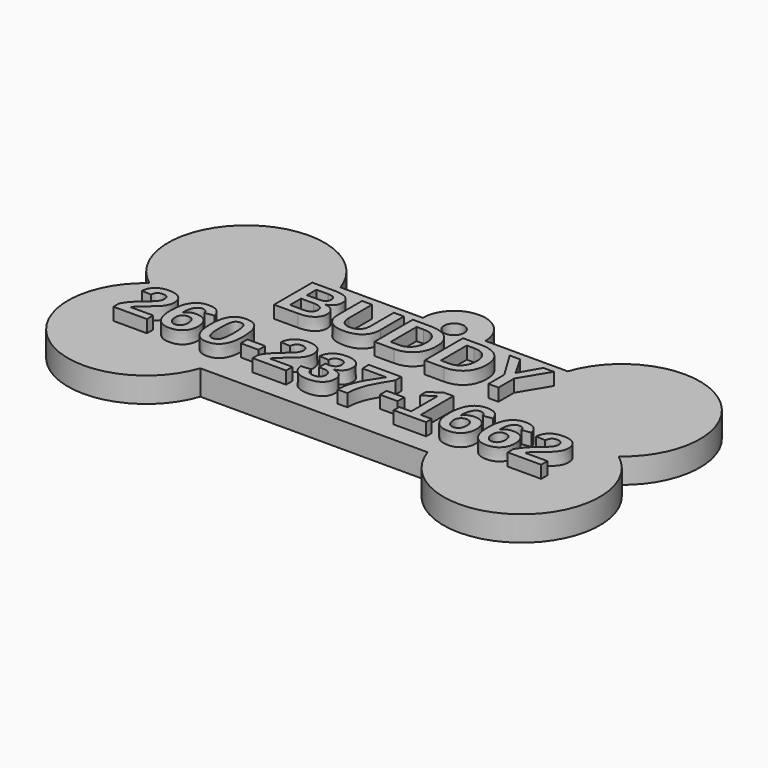
from build123d import *

# Parameters (mm, degrees)
F0_R         = 1.016
F1_DEPTH     = 2.54
F2_TEXT_SIZE = 7.0555555556
F3_DEPTH     = 1.27
F4_TEXT_SIZE = 7.0555555556
F5_DEPTH     = 1.27


# Not quite as in the source:
# - Text() gives the source's letters only with a copy of the font that has no kerning and outlines rounded to 1/6400 em; it was checked with that copy


with BuildPart() as f1:
    # F0 (on Top) → F1 (new body)
    with BuildSketch(Plane.XY):
        with BuildLine():
            Line((-15.2811150611, 27.291036626), (-23.6359883168, 27.291036626))
            ThreePointArc((-23.6359883168, 27.291036626), (-35.8100543941, 31.1810253456), (-35.9186150611, 18.401036626))
            ThreePointArc((-35.9186150611, 18.401036626), (-35.8100543941, 5.6210479063), (-23.6359883168, 9.511036626))
            Line((-23.6359883168, 9.511036626), (-0.5762418054, 9.511036626))
            ThreePointArc((-0.5762418054, 9.511036626), (11.5978242719, 5.6210479063), (11.7063849389, 18.401036626))
            ThreePointArc((11.7063849389, 18.401036626), (11.5978242719, 31.1810253456), (-0.5762418054, 27.291036626))
            Line((-0.5762418054, 27.291036626), (-8.9311150611, 27.291036626))
            ThreePointArc((-8.9311150611, 27.291036626), (-12.1061150611, 30.466036626), (-15.2811150611, 27.291036626))
        make_face()
        with Locations((-12.1061150611, 27.291036626)):
            Circle(F0_R, mode=Mode.SUBTRACT)
    extrude(amount=-F1_DEPTH)

    # F2 (on face) → F3 (join)
    with BuildSketch(Plane.XY):
        with Locations((-24.8380855472, 19.781898944)):
            Text('BUDDY', F2_TEXT_SIZE, font='Arimo', font_style=FontStyle.BOLD, text_align=(TextAlign.LEFT, TextAlign.BOTTOM))
    extrude(amount=F3_DEPTH)

    # F4 (on face) → F5 (join)
    with BuildSketch(Plane.XY):
        with Locations((-34.3300638513, 11.5541539654)):
            Text('260-237-1662', F4_TEXT_SIZE, font='Arimo', font_style=FontStyle.BOLD, text_align=(TextAlign.LEFT, TextAlign.BOTTOM))
    extrude(amount=F5_DEPTH)


solid = f1.part
